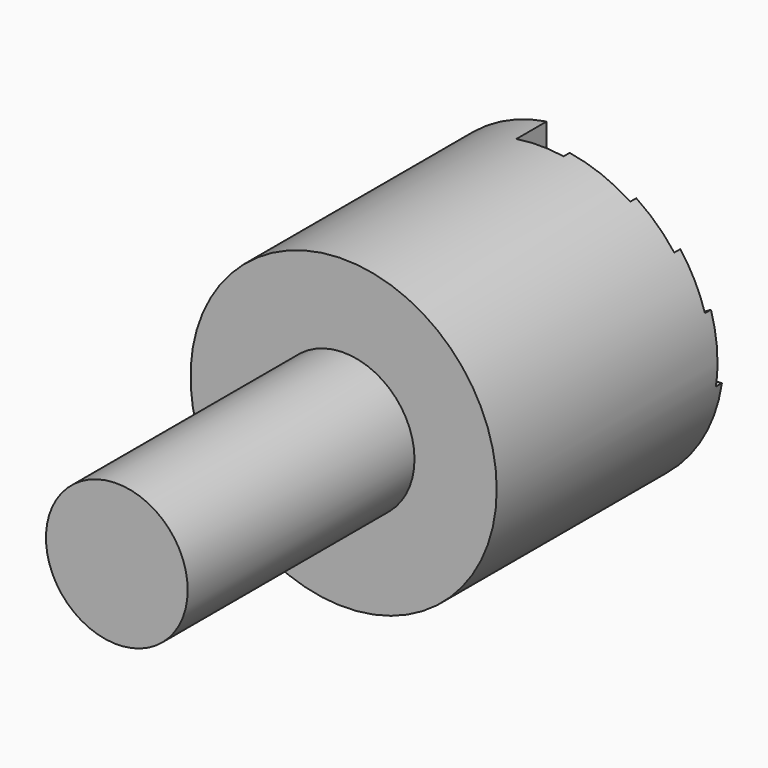
from build123d import *

# Parameters (mm, degrees)
F0_R      = 10.287
F1_DEPTH  = 38.1
F2_R      = 10.287
F2_R_2    = 4.7625
F3_DEPTH  = 19.05
F4_R      = 6.4135
F5_DEPTH  = 12.7
F7_DEPTH  = 2.54
F9_DEPTH  = 2.032
F11_DEPTH = 1.524
F13_DEPTH = 1.016
F15_DEPTH = 0.508


# Not quite as in the source:
# - a feature names something its author has since deleted; it is built from what else it names


with BuildPart() as f1:
    # F0 (on Front) → F1 (new body)
    with BuildSketch(Plane.XZ):
        Circle(F0_R)
    extrude(amount=F1_DEPTH)

    # F2 (on face) → F3 (cut)
    with BuildSketch(Plane.XZ.offset(38.1)):
        Circle(F2_R)
        Circle(F2_R_2, mode=Mode.SUBTRACT)
    extrude(amount=-F3_DEPTH, mode=Mode.SUBTRACT)

    # F4 (on face) → F5 (cut)
    with BuildSketch(Plane(origin=(0, 0, 0), x_dir=(-1, 0, 0), z_dir=(0, 1, 0))):
        Circle(F4_R)
    extrude(amount=-F5_DEPTH, mode=Mode.SUBTRACT)

    # F6 (on face) → F7 (cut)
    with BuildSketch(Plane(origin=(0, 0, 0), x_dir=(-1, 0, 0), z_dir=(0, 1, 0))):
        with BuildLine():
            ThreePointArc((1.6002, 10.1617778445), (0.0128539811, 10.2869919692), (-1.5748, 10.1657451257))
            Line((-1.5748, 10.1657451257), (-1.5748, 6.217152661))
            ThreePointArc((-1.5748, 6.217152661), (0.013107899, 6.413486605), (1.6002, 6.2106635885))
            Line((1.6002, 6.2106635885), (1.6002, 10.1617778445))
        make_face()
        with BuildLine():
            Line((-1.5748, -6.217152661), (-1.5748, -10.1657451257))
            ThreePointArc((-1.5748, -10.1657451257), (0.0128539811, -10.2869919692), (1.6002, -10.1617778445))
            Line((1.6002, -10.1617778445), (1.6002, -6.2106635885))
            ThreePointArc((1.6002, -6.2106635885), (0.013107899, -6.413486605), (-1.5748, -6.217152661))
        make_face()
    extrude(amount=-F7_DEPTH, mode=Mode.SUBTRACT)

    # F8 (on face) → F9 (cut)
    with BuildSketch(Plane(origin=(0, 0, 0), x_dir=(-1, 0, 0), z_dir=(0, 1, 0))):
        with BuildLine():
            ThreePointArc((-1.5748, 10.1657451257), (-3.6933269708, 9.6011303963), (-5.6440857783, 8.6003874754))
            Line((-5.6440857783, 8.6003874754), (-4.2590825341, 4.795122336))
            ThreePointArc((-4.2590825341, 4.795122336), (-3.0023472345, 5.6673532917), (-1.5748, 6.217152661))
            Line((-1.5748, 6.217152661), (-1.5748, 10.1657451257))
        make_face()
        with BuildLine():
            Line((-1.6895483294, 11.5486066381), (-6.129032147, 9.932766673))
            Line((-6.129032147, 9.932766673), (-5.6440857783, 8.6003874754))
            ThreePointArc((-5.6440857783, 8.6003874754), (-3.6933269708, 9.6011303963), (-1.5748, 10.1657451257))
            Line((-1.5748, 10.1657451257), (-1.5748, 6.217152661))
            ThreePointArc((-1.5748, 6.217152661), (-3.0023472345, 5.6673532917), (-4.2590825341, 4.795122336))
            Line((-4.2590825341, 4.795122336), (1.6895483294, -11.5486066381))
            Line((1.6895483294, -11.5486066381), (6.129032147, -9.932766673))
            Line((6.129032147, -9.932766673), (-1.6895483294, 11.5486066381))
        make_face()
    extrude(amount=-F9_DEPTH, mode=Mode.SUBTRACT)

    # F10 (on face) → F11 (cut)
    with BuildSketch(Plane(origin=(0, 0, 0), x_dir=(-1, 0, 0), z_dir=(0, 1, 0))):
        with BuildLine():
            ThreePointArc((-5.6440857783, 8.6003874754), (-7.0232543947, 7.5163998502), (-8.1981986695, 6.213848049))
            Line((-8.1981986695, 6.213848049), (-5.6029284192, 3.1209254044))
            ThreePointArc((-5.6029284192, 3.1209254044), (-5.0015546435, 4.0146523384), (-4.2590825341, 4.795122336))
            Line((-4.2590825341, 4.795122336), (-5.6440857783, 8.6003874754))
        make_face()
        with BuildLine():
            Line((-5.5958847817, 10.2253004606), (-9.0982399757, 7.2864755091))
            Line((-9.0982399757, 7.2864755091), (-8.1981986695, 6.213848049))
            ThreePointArc((-8.1981986695, 6.213848049), (-7.0232543947, 7.5163998502), (-5.6440857783, 8.6003874754))
            Line((-5.6440857783, 8.6003874754), (-4.2590825341, 4.795122336))
            ThreePointArc((-4.2590825341, 4.795122336), (-5.0015546435, 4.0146523384), (-5.6029284192, 3.1209254044))
            Line((-5.6029284192, 3.1209254044), (5.5958847817, -10.2253004606))
            Line((5.5958847817, -10.2253004606), (9.0982399757, -7.2864755091))
            Line((9.0982399757, -7.2864755091), (-5.5958847817, 10.2253004606))
        make_face()
    extrude(amount=-F11_DEPTH, mode=Mode.SUBTRACT)

    # F12 (on face) → F13 (cut)
    with BuildSketch(Plane(origin=(0, 0, 0), x_dir=(-1, 0, 0), z_dir=(0, 1, 0))):
        with BuildLine():
            Line((-14.7145799005, 11.2231002783), (-17.0767799005, 7.1316498607))
            Line((-17.0767799005, 7.1316498607), (15.3816246724, -11.6082187569))
            Line((15.3816246724, -11.6082187569), (17.7438246724, -7.5167683393))
            Line((17.7438246724, -7.5167683393), (9.8518430547, -2.9603306279))
            ThreePointArc((9.8518430547, -2.9603306279), (9.1704604826, -4.6610109994), (8.1981986695, -6.213848049))
            Line((8.1981986695, -6.213848049), (5.6029284192, -3.1209254044))
            ThreePointArc((5.6029284192, -3.1209254044), (6.0730159591, -2.0619067413), (6.3448917326, -0.935591338))
            Line((6.3448917326, -0.935591338), (-14.7145799005, 11.2231002783))
        make_face()
        with BuildLine():
            Line((9.8518430547, -2.9603306279), (6.3448917326, -0.935591338))
            ThreePointArc((6.3448917326, -0.935591338), (6.0730159591, -2.0619067413), (5.6029284192, -3.1209254044))
            Line((5.6029284192, -3.1209254044), (8.1981986695, -6.213848049))
            ThreePointArc((8.1981986695, -6.213848049), (9.1704604826, -4.6610109994), (9.8518430547, -2.9603306279))
        make_face()
    extrude(amount=-F13_DEPTH, mode=Mode.SUBTRACT)

    # F14 (on face) → F15 (cut)
    with BuildSketch(Plane(origin=(0, 0, 0), x_dir=(-1, 0, 0), z_dir=(0, 1, 0))):
        with BuildLine():
            Line((-25.8091024604, 4.6292271013), (-26.2208610514, -0.0771951304))
            Line((-26.2208610514, -0.0771951304), (-10.1798918612, -1.4805980865))
            ThreePointArc((-10.1798918612, -1.4805980865), (-10.260188024, -0.7422335965), (-10.287, 0))
            ThreePointArc((-10.287, 0), (-10.1776293532, 1.4960714382), (-9.8518430547, 2.9603306279))
            Line((-9.8518430547, 2.9603306279), (-6.3448917326, 0.935591338))
            ThreePointArc((-6.3448917326, 0.935591338), (-6.3969914921, -0.4598718295), (-6.1458227701, -1.8335333998))
            Line((-6.1458227701, -1.8335333998), (22.5503757634, -4.3441254578))
            Line((22.5503757634, -4.3441254578), (22.9621343545, 0.3622967739))
            Line((22.9621343545, 0.3622967739), (-25.8091024604, 4.6292271013))
        make_face()
        with BuildLine():
            ThreePointArc((-10.287, 0), (-10.260188024, -0.7422335965), (-10.1798918612, -1.4805980865))
            Line((-10.1798918612, -1.4805980865), (-6.1458227701, -1.8335333998))
            ThreePointArc((-6.1458227701, -1.8335333998), (-6.3969914921, -0.4598718295), (-6.3448917326, 0.935591338))
            Line((-6.3448917326, 0.935591338), (-9.8518430547, 2.9603306279))
            ThreePointArc((-9.8518430547, 2.9603306279), (-10.1776293532, 1.4960714382), (-10.287, 0))
        make_face()
    extrude(amount=-F15_DEPTH, mode=Mode.SUBTRACT)


solid = f1.part
